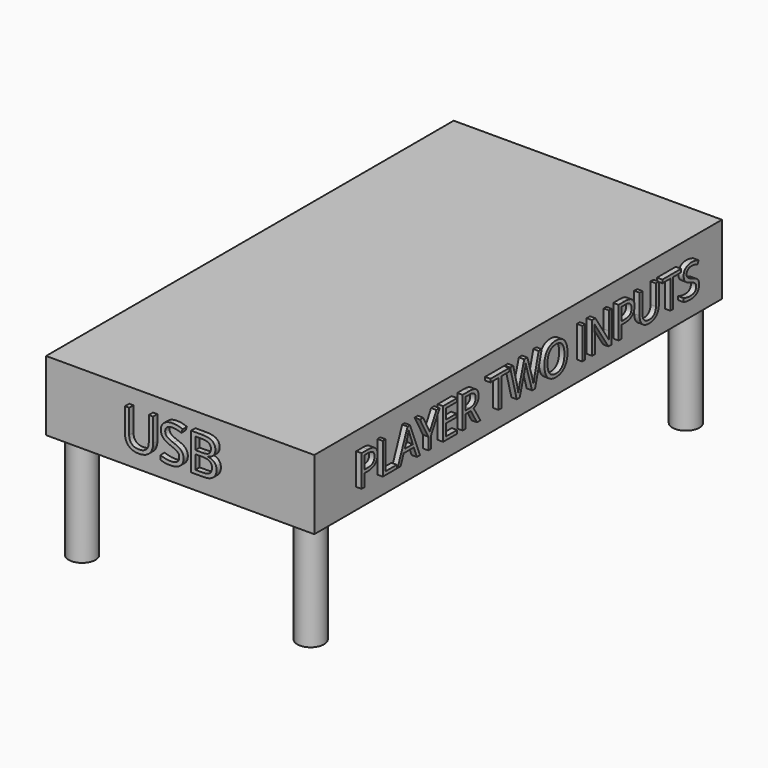
from build123d import *

# Parameters (mm, degrees)
F0_W         = 50
F0_H         = 95
F1_DEPTH     = 13
F2_TEXT_SIZE = 9.6051695032
F3_DEPTH     = 1
F4_TEXT_SIZE = 7.4362595721
F5_DEPTH     = 1
F6_TEXT_SIZE = 8.2073641858
F7_DEPTH     = 1
F8_R         = 2.5
F9_DEPTH     = 20


# Not quite as in the source:
# - Text() gives the source's letters only with a copy of the font that has no kerning and outlines rounded to 1/6400 em; it was checked with that copy


with BuildPart() as f1:
    # F0 (on Top) → F1 (new body)
    with BuildSketch(Plane.XY):
        Rectangle(F0_W, F0_H)
    extrude(amount=F1_DEPTH)

    # F2 (on face) → F3 (join)
    with BuildSketch(Plane.XZ.offset(47.5)):
        with Locations((-10.3735839948, 3.3463174477)):
            Text('USB', F2_TEXT_SIZE, font='Open Sans', text_align=(TextAlign.LEFT, TextAlign.BOTTOM))
    extrude(amount=F3_DEPTH)

    # F4 (on face) → F5 (join)
    with BuildSketch(Plane(origin=(-25, 0, 0), x_dir=(0, -1, 0), z_dir=(-1, 0, 0))):
        with Locations((-36.0286831856, 4.6848445199)):
            Text('PLAYER ONE INPUTS', F4_TEXT_SIZE, font='Open Sans', text_align=(TextAlign.LEFT, TextAlign.BOTTOM))
    extrude(amount=F5_DEPTH)

    # F6 (on face) → F7 (join)
    with BuildSketch(Plane.YZ.offset(25)):
        with Locations((-38.5245811385, 3.7924452146)):
            Text('PLAYER TWO INPUTS', F6_TEXT_SIZE, font='Open Sans', text_align=(TextAlign.LEFT, TextAlign.BOTTOM))
    extrude(amount=F7_DEPTH)

    # F8 (on face) → F9 (join)
    with BuildSketch(Plane(origin=(0, 0, 0), x_dir=(1, 0, 0), z_dir=(0, 0, -1))):
        with Locations((-21.3048867881, 43.7252148986)):
            Circle(F8_R)
        with Locations((21.3048867881, 43.7252148986)):
            Circle(F8_R)
        with Locations((21.3048867881, -43.7252148986)):
            Circle(F8_R)
        with Locations((-21.3048867881, -43.7252148986)):
            Circle(F8_R)
    extrude(amount=F9_DEPTH)


solid = f1.part
